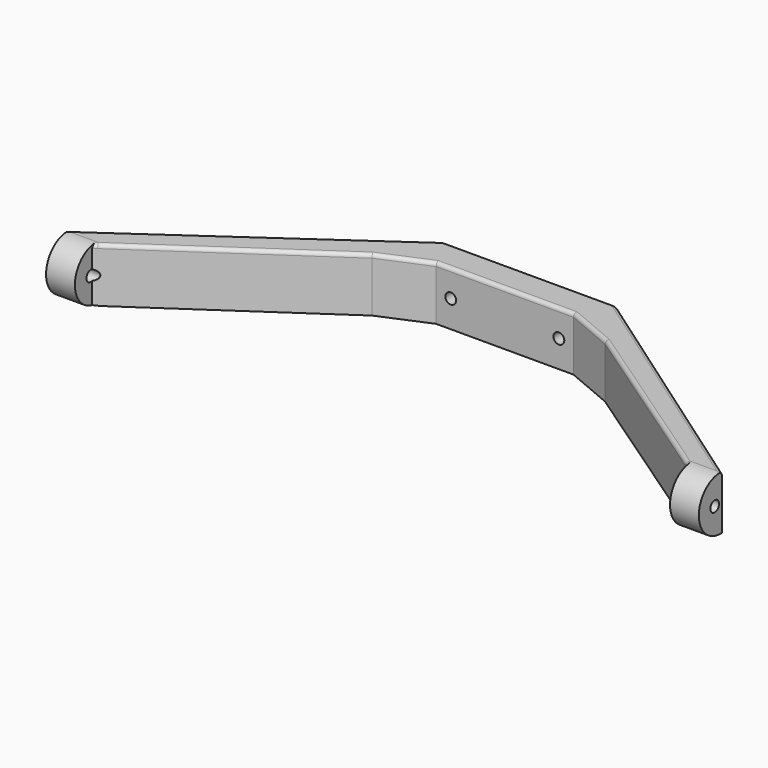
from build123d import *

# Parameters (mm, degrees)
F1_DEPTH    = 15
F3_D        = 3
F5_D        = 3
F6_T1_DEPTH = 45.5
F6_T3_DEPTH = 45.5
F7_T1_DEPTH = 85
F7_T3_DEPTH = 85
F8_SIZE2    = 10
F8_SIZE     = 5
F9_R        = 1


# Not quite as in the source:
# - a fillet or chamfer that OpenCascade refuses, or shapes differently, is made with other operations: its cross-section is extruded or revolved along the edge and cut away or added
# - a feature names something its author has since deleted; it is built from what else it names


with BuildPart() as f1:
    # F0 (on Top) → F1 (new body)
    with BuildSketch(Plane.XY):
        Polygon((20.4625322646, 0), (-29.5374677354, 0), (-95.0696312785, -45.8861149081), (-95.0696312785, -53.8861149081), (-87.0696312785, -53.8861149081), (-87.0696312785, -47.8861149081), (-28.5915713688, -8), (19.516635898, -8), (77.9946958077, -47.8861149081), (77.9946958077, -53.8861149081), (85.9946958077, -53.8861149081), (85.9946958077, -45.8861149081), align=None)
    extrude(amount=F1_DEPTH)

    # F3 (through all)
    with Locations(Plane.XZ.offset(8)):
        with Locations((10.4625322646, 7.5), (-19.5374677354, 7.5)):
            Hole(F3_D / 2)

    # F5 (through all)
    with Locations(Plane.YZ.offset(85.9946958077)):
        with Locations((-48.3861149081, 7.5)):
            Hole(F5_D / 2)

    # F6: fillet of radius 7.5 on 4 edges, made by hand

    # F6_s2 → F6_t1 (cut)
    with BuildSketch(Plane.YZ.offset(59.2446958077)):
        with BuildLine():
            ThreePointArc((-46.3861149081, 0), (-51.689415767, 2.1966991411), (-53.8861149081, 7.5))
            Line((-53.8861149081, 7.5), (-53.8861149081, 0))
            Line((-53.8861149081, 0), (-46.3861149081, 0))
        make_face()
        with BuildLine():
            ThreePointArc((-46.3861149081, 15), (-51.689415767, 12.8033008589), (-53.8861149081, 7.5))
            Line((-53.8861149081, 7.5), (-53.8861149081, 15))
            Line((-53.8861149081, 15), (-46.3861149081, 15))
        make_face()
    extrude(amount=F6_T1_DEPTH, mode=Mode.SUBTRACT)

    # F6_s4 → F6_t3 (cut)
    with BuildSketch(Plane.YZ.offset(-113.8196312785)):
        with BuildLine():
            ThreePointArc((-46.3861149081, 0), (-51.689415767, 2.1966991411), (-53.8861149081, 7.5))
            Line((-53.8861149081, 7.5), (-53.8861149081, 0))
            Line((-53.8861149081, 0), (-46.3861149081, 0))
        make_face()
        with BuildLine():
            ThreePointArc((-46.3861149081, 15), (-51.689415767, 12.8033008589), (-53.8861149081, 7.5))
            Line((-53.8861149081, 7.5), (-53.8861149081, 15))
            Line((-53.8861149081, 15), (-46.3861149081, 15))
        make_face()
    extrude(amount=F6_T3_DEPTH, mode=Mode.SUBTRACT)

    # F7: fillet of radius 1 on 2 edges, made by hand

    # F7_s2 → F7_t1 (cut)
    with BuildSketch(Plane(origin=(-17.7720582311, -12.4441291429, 0), x_dir=(0, 0, 1), z_dir=(-0.8191520443, -0.5735764364, 0))):
        with BuildLine():
            ThreePointArc((14, 16.9419954825), (14.7071067812, 16.6491022637), (15, 15.9419954825))
            Line((15, 15.9419954825), (15, 16.9419954825))
            Line((15, 16.9419954825), (14, 16.9419954825))
        make_face()
    extrude(amount=F7_T1_DEPTH, mode=Mode.SUBTRACT)

    # F7_s4 → F7_t3 (cut)
    with BuildSketch(Plane(origin=(81.3106088951, -56.9343012848, 0), x_dir=(0, 0, 1), z_dir=(-0.8191520443, 0.5735764364, 0))):
        with BuildLine():
            ThreePointArc((15, 10.7368263351), (14.7071067812, 11.4439331162), (14, 11.7368263351))
            Line((14, 11.7368263351), (15, 11.7368263351))
            Line((15, 11.7368263351), (15, 10.7368263351))
        make_face()
    extrude(amount=F7_T3_DEPTH, mode=Mode.SUBTRACT)

    # F8
    f8_edges = [f1.edges().sort_by_distance(p)[0] for p in [
        (-28.591571, -8, 7.5),
        (19.516636, -8, 7.5),
    ]]
    f8_side = f1.faces().sort_by_distance((-4.537468, -8, 7.5))[0]
    chamfer(f8_edges, length=F8_SIZE, length2=F8_SIZE2, reference=f8_side)

    # F9
    f9_edges = [f1.edges().sort_by_distance(p)[0] for p in [
        (-60.86166, -30.010451, 15),
        (-30.222224, -10.817393, 15),
        (-4.537468, -8, 15),
        (21.147289, -10.817393, 15),
        (51.786725, -30.010451, 15),
    ]]
    fillet(f9_edges, radius=F9_R)


solid = f1.part
